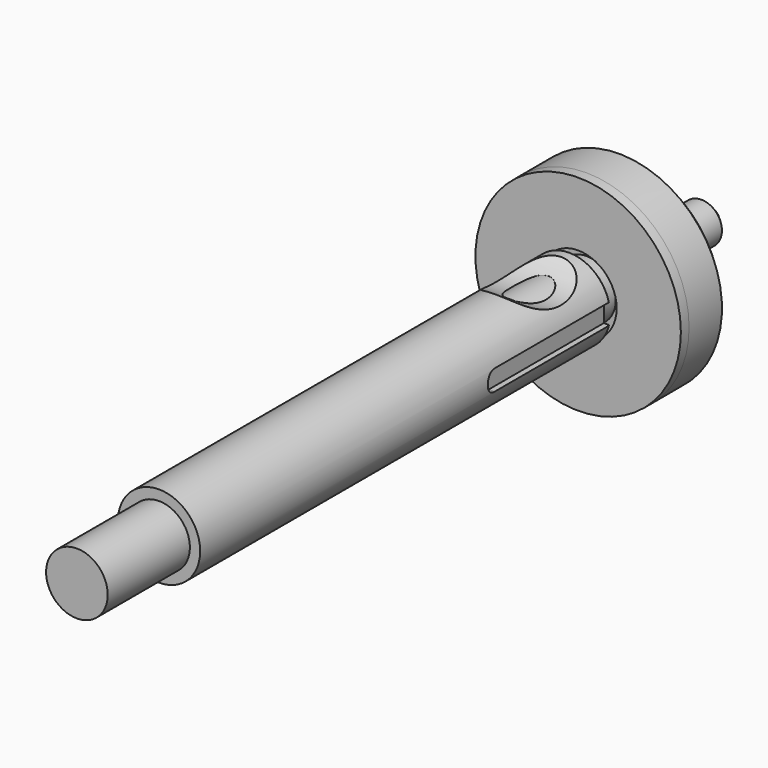
from build123d import *

# Parameters (mm, degrees)
F0_R          = 4
F0_R_2        = 3
F1_DEPTH      = 50
F2_R          = 6
F3_DEPTH      = 25
F3_DEPTH_BACK = 25
F5_DEPTH      = 15
F6_SIZE       = 0.1
F7_R          = 0.9999
F8_R          = 3
F9_DEPTH      = 2
F9_DEPTH_BACK = 60
F12_R         = 2
F13_DEPTH     = 15
F14_SIZE      = 1
F15_R         = 10
F16_DEPTH     = 5
F17_R         = 10
F17_R_2       = 3.75
F18_DEPTH     = 1
F20_SIZE      = 1


# Not quite as in the source:
# - a fillet or chamfer that OpenCascade refuses, or shapes differently, is made with other operations: its cross-section is extruded or revolved along the edge and cut away or added
# - a fillet or chamfer is up to 0.001 mm smaller than in the source, because OpenCascade refuses the exact size


with BuildPart() as f1:
    # F0 (on Front) → F1 (new body)
    with BuildSketch(Plane.XZ):
        Circle(F0_R)
        Circle(F0_R_2, mode=Mode.SUBTRACT)
    extrude(amount=F1_DEPTH)

    # F2 (on Right) → F3 (cut, two sides)
    with BuildSketch(Plane.YZ) as f3_sk:
        with Locations((-5, 8.5)):
            Circle(F2_R)
    extrude(amount=-F3_DEPTH, mode=Mode.SUBTRACT)
    extrude(f3_sk.sketch, amount=F3_DEPTH_BACK, mode=Mode.SUBTRACT)

    # F4 (on face) → F5 (cut)
    with BuildSketch(Plane(origin=(0, 0, 0), x_dir=(-1, 0, 0), z_dir=(0, 1, 0))):
        Polygon((-4.3, 1), (-4.3, 0), (-4.3, -1), (-3.3, -1), (-3.3, 1), align=None)
        Polygon((1, -3.3), (-1, -3.3), (-1, -4.3), (0, -4.3), (1, -4.3), align=None)
        Polygon((3.3, 1), (3.3, -1), (4.3, -1), (4.3, 0), (4.3, 1), align=None)
    extrude(amount=-F5_DEPTH, mode=Mode.SUBTRACT)

    # F6
    f6_edges = [f1.edges().sort_by_distance(p)[0] for p in [
        (0, 0, 4),
        (2.828427, 0, -2.828427),
        (-2.828427, 0, -2.828427),
    ]]
    chamfer(f6_edges, length=F6_SIZE)

    # F7 (radius 1 in the source; OpenCascade refuses exactly that, so slightly less here)
    f7_edges = [f1.edges().sort_by_distance(p)[0] for p in [
        (3.586492, -15, 1),
        (3.586492, -15, -1),
        (1, -15, -3.586492),
        (-1, -15, -3.586492),
        (-3.586492, -15, -1),
        (-3.586492, -15, 1),
    ]]
    fillet(f7_edges, radius=F7_R)

    # F8 (on face) → F9 (join, two sides)
    with BuildSketch(Plane(origin=(0, 0, 0), x_dir=(-1, 0, 0), z_dir=(0, 1, 0))) as f9_sk:
        Circle(F8_R)
    extrude(amount=F9_DEPTH)
    extrude(f9_sk.sketch, amount=-F9_DEPTH_BACK)

    # F10: chamfer of 2 x 0.1398536239 on 1 edges, made by hand


with BuildPart() as f10_tool2:
    # F10_s3 → F10_t4 (revolve)
    with BuildSketch(Plane.XY):
        Polygon((-3, 0), (-2.8601463761, 2), (-3, 2), align=None)
    revolve(axis=Axis((0, 2, 0), (0, 1, 0)))

    split(bisect_by=Plane.XZ, keep=Keep.BOTTOM)


with BuildPart() as f1_1:
    add(f1.part)

    # F10_t1: cut F10_tool2
    add(f10_tool2.part, mode=Mode.SUBTRACT)

    # F12 (on face) → F13 (join)
    with BuildSketch(Plane(origin=(0, 2, 0), x_dir=(-1, 0, 0), z_dir=(0, 1, 0))):
        Circle(F12_R)
    extrude(amount=F13_DEPTH)

    # F14
    f14_edges = [f1_1.edges().sort_by_distance(p)[0] for p in [
        (2, 17, 0),
    ]]
    chamfer(f14_edges, length=F14_SIZE)

    # F15 (on face) → F16 (join)
    with BuildSketch(Plane(origin=(0, 2, 0), x_dir=(-1, 0, 0), z_dir=(0, 1, 0))):
        Circle(F15_R)
    extrude(amount=F16_DEPTH)

    # F17 (on face) → F18 (join)
    with BuildSketch(Plane.XZ.offset(-2)):
        Circle(F17_R)
        Circle(F17_R_2, mode=Mode.SUBTRACT)
    extrude(amount=F18_DEPTH)

    # F20
    f20_edges = [f1_1.edges().sort_by_distance(p)[0] for p in [
        (10, 7, 0),
    ]]
    chamfer(f20_edges, length=F20_SIZE)


solid = f1_1.part
